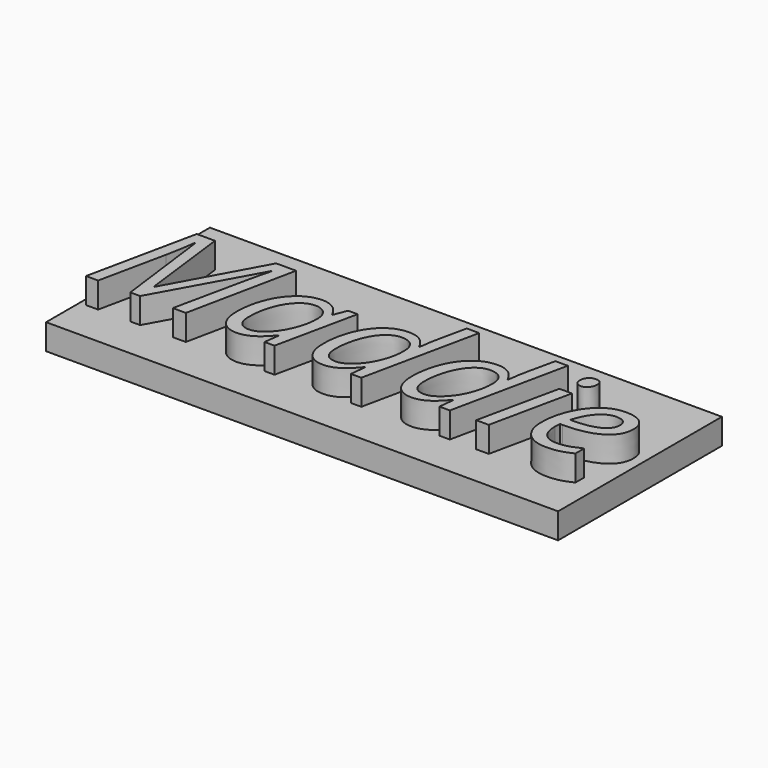
from build123d import *

# Parameters (mm, degrees)
F0_W         = 63.5
F0_H         = 25.4
F1_DEPTH     = 3.175
F2_TEXT_SIZE = 19.0235453822
F3_DEPTH     = 3.175


# Not quite as in the source:
# - Text() gives the source's letters only with a copy of the font that has no kerning and outlines rounded to 1/6400 em; it was checked with that copy


with BuildPart() as f1:
    # F0 (on Top) → F1 (new body)
    with BuildSketch(Plane.XY):
        with Locations((31.75, 12.7)):
            Rectangle(F0_W, F0_H)
    extrude(amount=F1_DEPTH)

    # F2 (on face) → F3 (join)
    with BuildSketch(Plane.XY.offset(3.175)):
        with Locations((0, 5.2085137154)):
            Text('Maddie', F2_TEXT_SIZE, font='Open Sans', font_style=FontStyle.ITALIC, text_align=(TextAlign.LEFT, TextAlign.BOTTOM))
    extrude(amount=F3_DEPTH)


solid = f1.part
